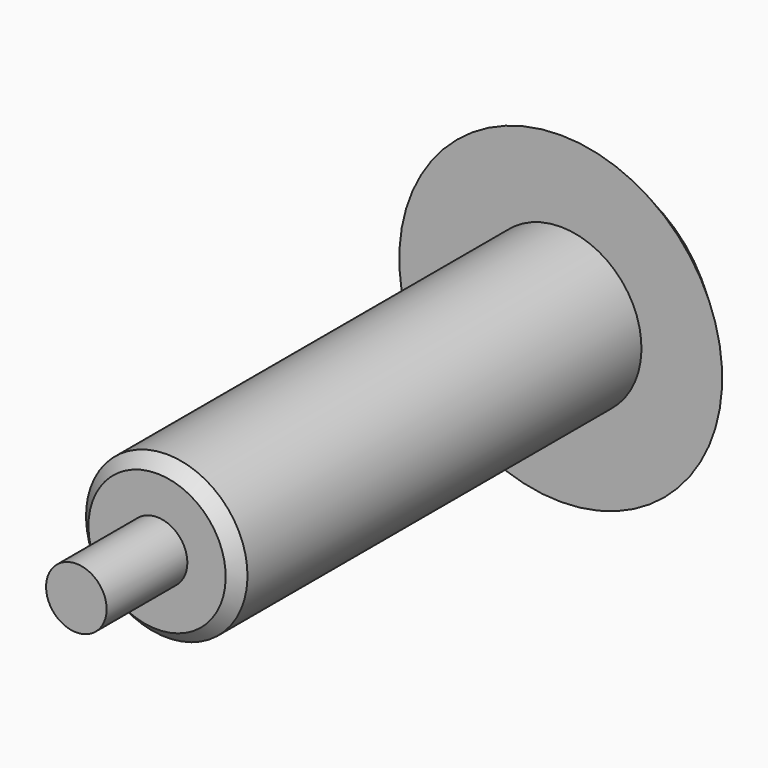
from build123d import *

# Parameters (mm, degrees)
F2_SIZE2 = 9.99999
F2_SIZE  = 9.99999
F3_SIZE2 = 3
F3_SIZE  = 3


# Not quite as in the source:
# - a fillet or chamfer is up to 0.001 mm smaller than in the source, because OpenCascade refuses the exact size


with BuildPart() as f1:
    # F0 (on Right) → F1 (revolve)
    with BuildSketch(Plane.YZ):
        Polygon((0, 0), (160, 0), (160, 40), (150, 40), (150, 20), (25, 20), (25, 7.5), (0, 7.5), align=None)
    revolve(axis=Axis((0, 80, 0), (0, 1, 0)))

    # F2 (size 10 and 10 in the source; OpenCascade refuses exactly that, so slightly less here)
    f2_edges = [f1.edges().sort_by_distance(p)[0] for p in [
        (0, 160, -40),
    ]]
    chamfer(f2_edges, length=F2_SIZE, length2=F2_SIZE2)

    # F3
    f3_edges = [f1.edges().sort_by_distance(p)[0] for p in [
        (0, 25, -20),
    ]]
    chamfer(f3_edges, length=F3_SIZE, length2=F3_SIZE2)


solid = f1.part
